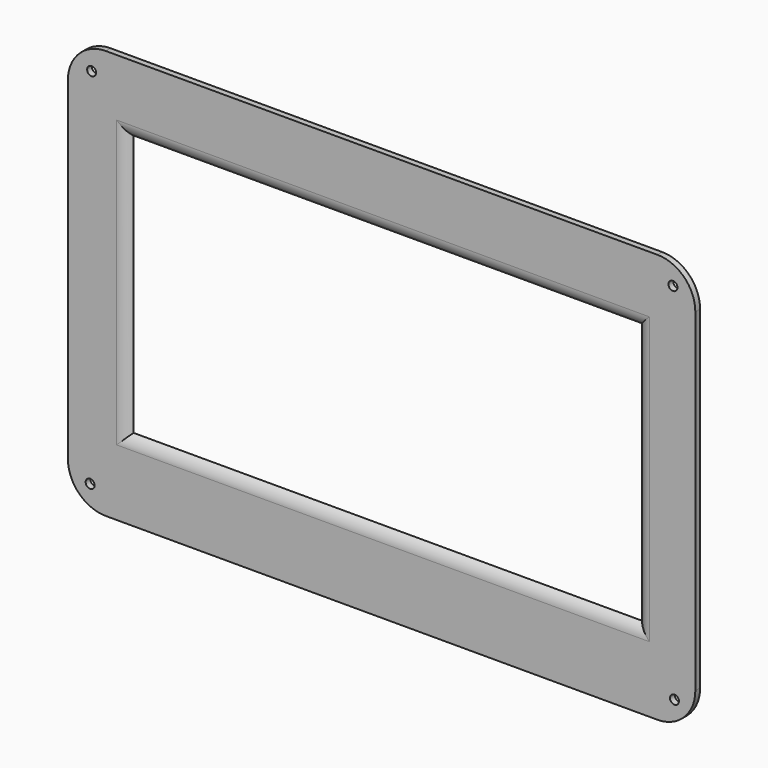
from build123d import *

# Parameters (mm, degrees)
F0_W         = 170.18
F0_H         = 87.63
F1_DEPTH     = 2
F3_D         = 3
F4_T1_DEPTH  = 87.63
F4_T3_DEPTH  = 170.18
F4_T9_DEPTH  = 97.7295049384
F4_T13_DEPTH = 180.2795049384
F4_T20_DEPTH = 97.7295049384
F4_T24_DEPTH = 180.2795049384
F4_T31_DEPTH = 180.2795049384
F4_T35_DEPTH = 97.7295049384
F4_T42_DEPTH = 180.2795049384
F4_T46_DEPTH = 97.7295049384


# Not quite as in the source:
# - a fillet or chamfer that OpenCascade refuses, or shapes differently, is made with other operations: its cross-section is extruded or revolved along the edge and cut away or added


with BuildPart() as f1:
    # F0 (on Front) → F1 (new body)
    with BuildSketch(Plane.XZ):
        with BuildLine():
            Line((94.3139557123, 80.8203592896), (-90.2860442877, 80.8203592896))
            ThreePointArc((-90.2860442877, 80.8203592896), (-99.2663004088, 77.1006154107), (-102.9860442877, 68.1203592896))
            Line((-102.9860442877, 68.1203592896), (-102.9860442877, -43.4872407104))
            ThreePointArc((-102.9860442877, -43.4872407104), (-99.2663004088, -52.4674968314), (-90.2860442877, -56.1872407104))
            Line((-90.2860442877, -56.1872407104), (94.3139557123, -56.1872407104))
            ThreePointArc((94.3139557123, -56.1872407104), (103.2942118334, -52.4674968314), (107.0139557123, -43.4872407104))
            Line((107.0139557123, -43.4872407104), (107.0139557123, 68.1203592896))
            ThreePointArc((107.0139557123, 68.1203592896), (103.2942118334, 77.1006154107), (94.3139557123, 80.8203592896))
        make_face()
        with Locations((2.4907932702, 13.8051814874)):
            Rectangle(F0_W, F0_H, mode=Mode.SUBTRACT)
    extrude(amount=F1_DEPTH)

    # F3 (through all)
    with Locations(Plane.XZ.offset(2)):
        with Locations((-95.5433249474, -48.3972094953), (-95.0444117188, 73.3367204666), (100.0292077661, -48.3972094953), (99.5303019881, 73.3367204666)):
            Hole(F3_D / 2)

    # F4: fillet of radius 5.08 on 4 edges, made by hand

    # F4_s2 → F4_t1 (cut)
    with BuildSketch(Plane.XY.offset(-30.0098185126)):
        with BuildLine():
            ThreePointArc((91.6205952456, -2), (89.3667097117, -1.4726256161), (87.5807932702, 0))
            Line((87.5807932702, 0), (87.5807932702, -2))
            Line((87.5807932702, -2), (91.6205952456, -2))
        make_face()
        with BuildLine():
            ThreePointArc((-86.6390087051, -2), (-84.3851231712, -1.4726256161), (-82.5992067298, 0))
            Line((-82.5992067298, 0), (-82.5992067298, -2))
            Line((-82.5992067298, -2), (-86.6390087051, -2))
        make_face()
    extrude(amount=F4_T1_DEPTH, mode=Mode.SUBTRACT)

    # F4_s4 → F4_t3 (cut)
    with BuildSketch(Plane.YZ.offset(-82.5992067298)):
        with BuildLine():
            ThreePointArc((-2, 61.6599834627), (-1.4726256161, 59.4060979288), (0, 57.6201814874))
            Line((0, 57.6201814874), (-2, 57.6201814874))
            Line((-2, 57.6201814874), (-2, 61.6599834627))
        make_face()
        with BuildLine():
            ThreePointArc((-2, -34.049620488), (-1.4726256161, -31.795734954), (0, -30.0098185126))
            Line((0, -30.0098185126), (-2, -30.0098185126))
            Line((-2, -30.0098185126), (-2, -34.049620488))
        make_face()
    extrude(amount=F4_T3_DEPTH, mode=Mode.SUBTRACT)


with BuildPart() as f4_tool7:
    # F4_s8 → F4_t9 (new body)
    with BuildSketch(Plane.XY.offset(67.7196864257)):
        with BuildLine():
            ThreePointArc((91.6205952456, -2), (89.3667097117, -1.4726256161), (87.5807932702, 0))
            Line((87.5807932702, 0), (87.5807932702, -2))
            Line((87.5807932702, -2), (91.6205952456, -2))
        make_face()
    extrude(amount=-F4_T9_DEPTH)

    split(bisect_by=Plane.XY.offset(57.6201814874), keep=Keep.TOP)


with BuildPart() as f4_tool11:
    # F4_s12 → F4_t13 (new body)
    with BuildSketch(Plane.YZ.offset(-82.5992067298)):
        with BuildLine():
            ThreePointArc((-2, 61.6599834627), (-1.4726256161, 59.4060979288), (0, 57.6201814874))
            Line((0, 57.6201814874), (-2, 57.6201814874))
            Line((-2, 57.6201814874), (-2, 61.6599834627))
        make_face()
    extrude(amount=F4_T13_DEPTH)

    split(bisect_by=Plane.YZ.offset(87.5807932702), keep=Keep.TOP)


with BuildPart() as f4_tool7_1:
    add(f4_tool7.part)

    # F4_t15: intersect F4_tool11
    add(f4_tool11.part, mode=Mode.INTERSECT)


with BuildPart() as f1_1:
    add(f1.part)

    # F4_t5: cut F4_tool7
    add(f4_tool7_1.part, mode=Mode.SUBTRACT)


with BuildPart() as f4_tool18:
    # F4_s19 → F4_t20 (new body)
    with BuildSketch(Plane.XY.offset(57.6201814874)):
        with BuildLine():
            ThreePointArc((91.6205952456, -2), (89.3667097117, -1.4726256161), (87.5807932702, 0))
            Line((87.5807932702, 0), (87.5807932702, -2))
            Line((87.5807932702, -2), (91.6205952456, -2))
        make_face()
    extrude(amount=-F4_T20_DEPTH)

    split(bisect_by=Plane.XY.offset(-30.0098185126), keep=Keep.BOTTOM)


with BuildPart() as f4_tool22:
    # F4_s23 → F4_t24 (new body)
    with BuildSketch(Plane.YZ.offset(97.6802982086)):
        with BuildLine():
            ThreePointArc((-2, -34.049620488), (-1.4726256161, -31.795734954), (0, -30.0098185126))
            Line((0, -30.0098185126), (-2, -30.0098185126))
            Line((-2, -30.0098185126), (-2, -34.049620488))
        make_face()
    extrude(amount=-F4_T24_DEPTH)

    split(bisect_by=Plane.YZ.offset(87.5807932702), keep=Keep.TOP)


with BuildPart() as f4_tool18_1:
    add(f4_tool18.part)

    # F4_t26: intersect F4_tool22
    add(f4_tool22.part, mode=Mode.INTERSECT)


with BuildPart() as f1_2:
    add(f1_1.part)

    # F4_t16: cut F4_tool18
    add(f4_tool18_1.part, mode=Mode.SUBTRACT)


with BuildPart() as f4_tool29:
    # F4_s30 → F4_t31 (new body)
    with BuildSketch(Plane.YZ.offset(-92.6987116681)):
        with BuildLine():
            ThreePointArc((-2, 61.6599834627), (-1.4726256161, 59.4060979288), (0, 57.6201814874))
            Line((0, 57.6201814874), (-2, 57.6201814874))
            Line((-2, 57.6201814874), (-2, 61.6599834627))
        make_face()
    extrude(amount=F4_T31_DEPTH)

    split(bisect_by=Plane.YZ.offset(-82.5992067298), keep=Keep.BOTTOM)


with BuildPart() as f4_tool33:
    # F4_s34 → F4_t35 (new body)
    with BuildSketch(Plane.XY.offset(-30.0098185126)):
        with BuildLine():
            ThreePointArc((-86.6390087051, -2), (-84.3851231712, -1.4726256161), (-82.5992067298, 0))
            Line((-82.5992067298, 0), (-82.5992067298, -2))
            Line((-82.5992067298, -2), (-86.6390087051, -2))
        make_face()
    extrude(amount=F4_T35_DEPTH)

    split(bisect_by=Plane.XY.offset(57.6201814874), keep=Keep.TOP)


with BuildPart() as f4_tool29_1:
    add(f4_tool29.part)

    # F4_t37: intersect F4_tool33
    add(f4_tool33.part, mode=Mode.INTERSECT)


with BuildPart() as f1_3:
    add(f1_2.part)

    # F4_t27: cut F4_tool29
    add(f4_tool29_1.part, mode=Mode.SUBTRACT)


with BuildPart() as f4_tool40:
    # F4_s41 → F4_t42 (new body)
    with BuildSketch(Plane.YZ.offset(87.5807932702)):
        with BuildLine():
            ThreePointArc((-2, -34.049620488), (-1.4726256161, -31.795734954), (0, -30.0098185126))
            Line((0, -30.0098185126), (-2, -30.0098185126))
            Line((-2, -30.0098185126), (-2, -34.049620488))
        make_face()
    extrude(amount=-F4_T42_DEPTH)

    split(bisect_by=Plane.YZ.offset(-82.5992067298), keep=Keep.BOTTOM)


with BuildPart() as f4_tool44:
    # F4_s45 → F4_t46 (new body)
    with BuildSketch(Plane.XY.offset(-40.109323451)):
        with BuildLine():
            ThreePointArc((-86.6390087051, -2), (-84.3851231712, -1.4726256161), (-82.5992067298, 0))
            Line((-82.5992067298, 0), (-82.5992067298, -2))
            Line((-82.5992067298, -2), (-86.6390087051, -2))
        make_face()
    extrude(amount=F4_T46_DEPTH)

    split(bisect_by=Plane.XY.offset(-30.0098185126), keep=Keep.BOTTOM)


with BuildPart() as f4_tool40_1:
    add(f4_tool40.part)

    # F4_t48: intersect F4_tool44
    add(f4_tool44.part, mode=Mode.INTERSECT)


with BuildPart() as f1_4:
    add(f1_3.part)

    # F4_t38: cut F4_tool40
    add(f4_tool40_1.part, mode=Mode.SUBTRACT)


solid = f1_4.part
